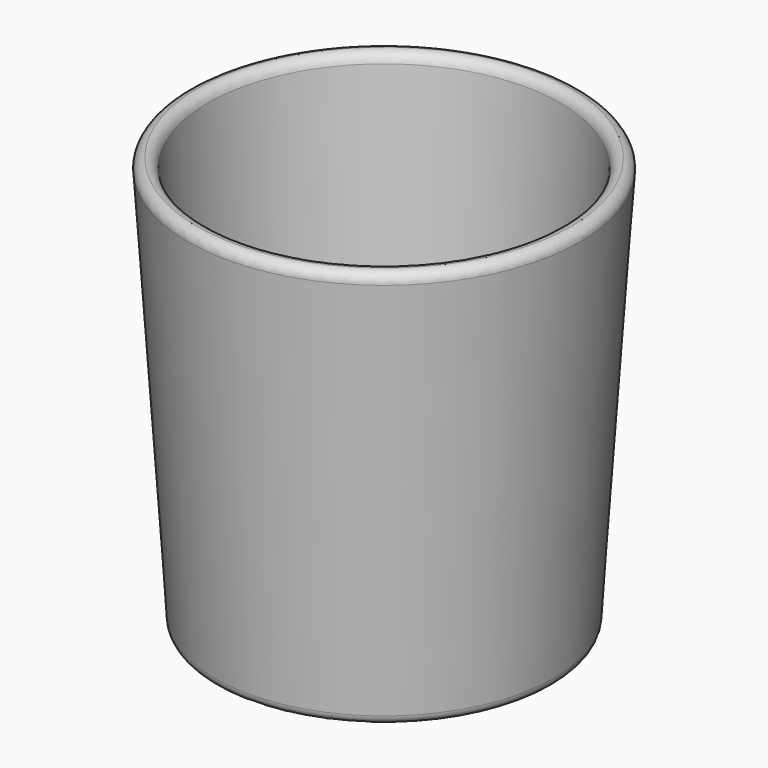
from build123d import *

# Parameters (mm, degrees)
F2_R = 2.4999


# Not quite as in the source:
# - a fillet or chamfer is up to 0.001 mm smaller than in the source, because OpenCascade refuses the exact size


with BuildPart() as f1:
    # F0 (on Front) → F1 (revolve)
    with BuildSketch(Plane.XZ):
        Polygon((0, 5), (0, 0), (42.9963162733, 0), (50, 104.666174073), (45.0111564215, 105), (38.3197073562, 5), align=None)
    revolve(axis=Axis((0, 0, 2.5), (0, 0, -1)))

    # F2 (radius 2.5 in the source; OpenCascade refuses exactly that, so slightly less here)
    f2_edges = [f1.edges().sort_by_distance(p)[0] for p in [
        (-50, 0, 104.666174),
        (-45.011156, 0, 105),
        (-42.996316, 0, 0),
        (-38.319707, 0, 5),
    ]]
    fillet(f2_edges, radius=F2_R)


solid = f1.part
